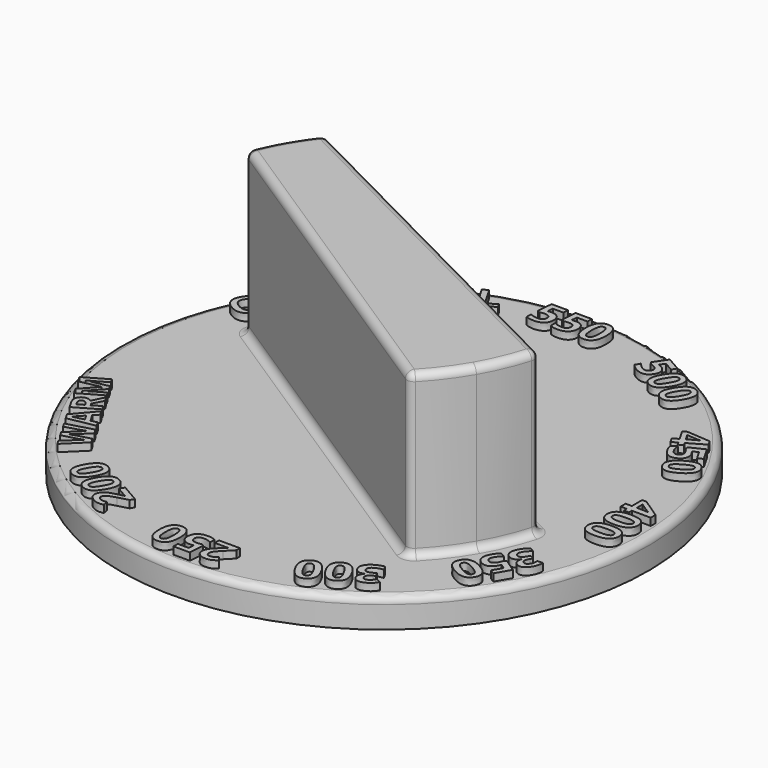
from build123d import *
from build123d import SkipClean  # not in build123d's __all__

# Parameters (mm, degrees)
F0_R          = 36
F0_R_2        = 5
F1_DEPTH      = 4
F2_DEPTH      = 26
F3_R          = 1
F4_DEPTH      = 25
F5_R          = 1
F6_DEPTH      = 4
F8_ANGLE      = -90
F9_TEXT_SIZE  = 5.2390307793
F10_DEPTH     = 1
F11_ANGLE     = 90
F12_TEXT_SIZE = 5.7419702135
F13_DEPTH     = 1
F14_ANGLE     = 30
F15_TEXT_SIZE = 5.7419702135
F16_DEPTH     = 1
F17_ANGLE     = 30
F18_TEXT_SIZE = 5.7419702135
F19_DEPTH     = 1
F20_ANGLE     = 30
F21_TEXT_SIZE = 5.7419702135
F22_DEPTH     = 1
F23_ANGLE     = 30
F24_TEXT_SIZE = 5.7419702135
F25_DEPTH     = 1
F26_ANGLE     = 30
F27_TEXT_SIZE = 5.7419702135
F28_DEPTH     = 1
F29_ANGLE     = 30
F30_TEXT_SIZE = 5.7419702135
F31_DEPTH     = 1
F32_ANGLE     = 60
F33_TEXT_SIZE = 5.2378516624
F34_DEPTH     = 1
F35_ANGLE     = 90
F36_TEXT_SIZE = 4.9233294015
F37_DEPTH     = 1
F38_ANGLE     = -120
F39_TEXT_SIZE = 5.7419702135
F40_DEPTH     = 1


# Not quite as in the source:
# - Text() gives the source's letters only with a copy of the font that has no kerning and outlines rounded to 1/6400 em; it was checked with that copy


with BuildPart() as f1:
    # F0 (on Top) → F1 (new body)
    with BuildSketch(Plane.XY):
        Circle(F0_R)
        with BuildLine():
            ThreePointArc((-26.2288567733, 6.6408985875), (-25.8537103282, 7.20647008), (-25.2038950976, 7.4022917703))
            Line((-25.2038950976, 7.4022917703), (27.7893484801, 4.5633680072))
            ThreePointArc((27.7893484801, 4.5633680072), (28.4145237228, 4.2992432559), (28.7270995296, 3.6968294999))
            ThreePointArc((28.7270995296, 3.6968294999), (28.9108711387, 1.8524734404), (28.9722179472, 0))
            ThreePointArc((28.9722179472, 0), (28.9108711387, -1.8524734404), (28.7270995296, -3.6968294999))
            ThreePointArc((28.7270995296, -3.6968294999), (28.4145237228, -4.2992432559), (27.7893484801, -4.5633680072))
            Line((27.7893484801, -4.5633680072), (-25.2038950976, -7.4022917703))
            ThreePointArc((-25.2038950976, -7.4022917703), (-25.8537103282, -7.20647008), (-26.2288567733, -6.6408985875))
            ThreePointArc((-26.2288567733, -6.6408985875), (-26.8273332377, -3.3443914115), (-27.0277820528, 0))
            ThreePointArc((-27.0277820528, 0), (-26.8273332377, 3.3443914115), (-26.2288567733, 6.6408985875))
        make_face(mode=Mode.SUBTRACT)
        with BuildLine():
            Line((27.7893484801, 4.5633680072), (-25.2038950976, 7.4022917703))
            ThreePointArc((-25.2038950976, 7.4022917703), (-25.8537103282, 7.20647008), (-26.2288567733, 6.6408985875))
            ThreePointArc((-26.2288567733, 6.6408985875), (-26.8273332377, 3.3443914115), (-27.0277820528, 0))
            ThreePointArc((-27.0277820528, 0), (-26.8273332377, -3.3443914115), (-26.2288567733, -6.6408985875))
            ThreePointArc((-26.2288567733, -6.6408985875), (-25.8537103282, -7.20647008), (-25.2038950976, -7.4022917703))
            Line((-25.2038950976, -7.4022917703), (27.7893484801, -4.5633680072))
            ThreePointArc((27.7893484801, -4.5633680072), (28.4145237228, -4.2992432559), (28.7270995296, -3.6968294999))
            ThreePointArc((28.7270995296, -3.6968294999), (28.9108711387, -1.8524734404), (28.9722179472, 0))
            ThreePointArc((28.9722179472, 0), (28.9108711387, 1.8524734404), (28.7270995296, 3.6968294999))
            ThreePointArc((28.7270995296, 3.6968294999), (28.4145237228, 4.2992432559), (27.7893484801, 4.5633680072))
        make_face()
        Circle(F0_R_2, mode=Mode.SUBTRACT)
        Circle(F0_R_2)
        with BuildLine():
            ThreePointArc((2.2360679775, 2), (0, -3), (-2.2360679775, 2))
            Line((-2.2360679775, 2), (2.2360679775, 2))
        make_face(mode=Mode.SUBTRACT)
        with BuildLine():
            Line((2.2360679775, 2), (-2.2360679775, 2))
            ThreePointArc((-2.2360679775, 2), (0, -3), (2.2360679775, 2))
        make_face()
    extrude(amount=F1_DEPTH)

    # F0 (on Top) → F2 (join)
    with BuildSketch(Plane.XY):
        with BuildLine():
            Line((27.7893484801, 4.5633680072), (-25.2038950976, 7.4022917703))
            ThreePointArc((-25.2038950976, 7.4022917703), (-25.8537103282, 7.20647008), (-26.2288567733, 6.6408985875))
            ThreePointArc((-26.2288567733, 6.6408985875), (-26.8273332377, 3.3443914115), (-27.0277820528, 0))
            ThreePointArc((-27.0277820528, 0), (-26.8273332377, -3.3443914115), (-26.2288567733, -6.6408985875))
            ThreePointArc((-26.2288567733, -6.6408985875), (-25.8537103282, -7.20647008), (-25.2038950976, -7.4022917703))
            Line((-25.2038950976, -7.4022917703), (27.7893484801, -4.5633680072))
            ThreePointArc((27.7893484801, -4.5633680072), (28.4145237228, -4.2992432559), (28.7270995296, -3.6968294999))
            ThreePointArc((28.7270995296, -3.6968294999), (28.9108711387, -1.8524734404), (28.9722179472, 0))
            ThreePointArc((28.9722179472, 0), (28.9108711387, 1.8524734404), (28.7270995296, 3.6968294999))
            ThreePointArc((28.7270995296, 3.6968294999), (28.4145237228, 4.2992432559), (27.7893484801, 4.5633680072))
        make_face()
        Circle(F0_R_2, mode=Mode.SUBTRACT)
        Circle(F0_R_2)
        with BuildLine():
            ThreePointArc((2.2360679775, 2), (0, -3), (-2.2360679775, 2))
            Line((-2.2360679775, 2), (2.2360679775, 2))
        make_face(mode=Mode.SUBTRACT)
        with BuildLine():
            Line((2.2360679775, 2), (-2.2360679775, 2))
            ThreePointArc((-2.2360679775, 2), (0, -3), (2.2360679775, 2))
        make_face()
    extrude(amount=F2_DEPTH)

    # F3
    f3_edges = [f1.edges().sort_by_distance(p)[0] for p in [
        (1.292727, 5.98283, 26),
        (28.414524, 4.299243, 26),
        (1.292727, -5.98283, 26),
        (-25.85371, 7.20647, 26),
        (-27.027782, 0, 26),
        (-25.85371, -7.20647, 26),
        (28.414524, -4.299243, 26),
        (28.972218, 0, 26),
    ]]
    fillet(f3_edges, radius=F3_R)

    # F0 (on Top) → F4 (cut)
    with BuildSketch(Plane.XY):
        with BuildLine():
            Line((2.2360679775, 2), (-2.2360679775, 2))
            ThreePointArc((-2.2360679775, 2), (0, -3), (2.2360679775, 2))
        make_face()
    extrude(amount=F4_DEPTH, mode=Mode.SUBTRACT)

    # F5
    f5_edges = [f1.edges().sort_by_distance(p)[0] for p in [
        (-36, 0, 4),
        (-25.85371, 7.20647, 4),
        (-27.027782, 0, 4),
        (-25.85371, -7.20647, 4),
        (1.292727, -5.98283, 4),
        (28.414524, -4.299243, 4),
        (28.972218, 0, 4),
        (28.414524, 4.299243, 4),
        (1.292727, 5.98283, 4),
    ]]
    fillet(f5_edges, radius=F5_R)

    # F0 (on Top) → F6 (join)
    with BuildSketch(Plane.XY):
        Circle(F0_R_2)
        with BuildLine():
            ThreePointArc((2.2360679775, 2), (0, -3), (-2.2360679775, 2))
            Line((-2.2360679775, 2), (2.2360679775, 2))
        make_face(mode=Mode.SUBTRACT)
    with SkipClean():  # cleaning this boolean's faces spoils the solid; the shape is the same uncleaned
        extrude(amount=-F6_DEPTH)


with BuildPart() as f1_1:
    # F8: moved
    add(f1.part.rotate(Axis((0, 0, 37.6716628671), (0, 0, -1)), F8_ANGLE), clean=False)

    # F9 (on face) → F10 (join)
    with BuildSketch(Plane.XY.offset(4)):
        with Locations((-4.9426552728, 30.7683626071)):
            Text('OFF', F9_TEXT_SIZE, font='Open Sans', font_style=FontStyle.BOLD, text_align=(TextAlign.LEFT, TextAlign.BOTTOM))
    extrude(amount=F10_DEPTH)


with BuildPart() as f1_2:
    # F11: moved
    add(f1_1.part.rotate(Axis((0, 0, 37.6716628671), (0, 0, -1)), F11_ANGLE), clean=False)

    # F12 (on face) → F13 (join)
    with BuildSketch(Plane.XY.offset(4)):
        with Locations((-5, 30.3274479291)):
            Text('200', F12_TEXT_SIZE, font='Open Sans', font_style=FontStyle.BOLD, text_align=(TextAlign.LEFT, TextAlign.BOTTOM))
    extrude(amount=F13_DEPTH)


with BuildPart() as f1_3:
    # F14: moved
    add(f1_2.part.rotate(Axis((0, 0, 37.6716628671), (0, 0, -1)), F14_ANGLE), clean=False)

    # F15 (on face) → F16 (join)
    with BuildSketch(Plane.XY.offset(4)):
        with Locations((-5, 30.5067975976)):
            Text('250', F15_TEXT_SIZE, font='Open Sans', font_style=FontStyle.BOLD, text_align=(TextAlign.LEFT, TextAlign.BOTTOM))
    extrude(amount=F16_DEPTH)


with BuildPart() as f1_4:
    # F17: moved
    add(f1_3.part.rotate(Axis((0, 0, 37.6716628671), (0, 0, -1)), F17_ANGLE), clean=False)

    # F18 (on face) → F19 (join)
    with BuildSketch(Plane.XY.offset(4)):
        with Locations((-5, 30.5067975976)):
            Text('300', F18_TEXT_SIZE, font='Open Sans', font_style=FontStyle.BOLD, text_align=(TextAlign.LEFT, TextAlign.BOTTOM))
    extrude(amount=F19_DEPTH)


with BuildPart() as f1_5:
    # F20: moved
    add(f1_4.part.rotate(Axis((0, 0, 37.6716628671), (0, 0, -1)), F20_ANGLE), clean=False)

    # F21 (on face) → F22 (join)
    with BuildSketch(Plane.XY.offset(4)):
        with Locations((-5, 30.5067975976)):
            Text('350', F21_TEXT_SIZE, font='Open Sans', font_style=FontStyle.BOLD, text_align=(TextAlign.LEFT, TextAlign.BOTTOM))
    extrude(amount=F22_DEPTH)


with BuildPart() as f1_6:
    # F23: moved
    add(f1_5.part.rotate(Axis((0, 0, 37.6716628671), (0, 0, -1)), F23_ANGLE), clean=False)

    # F24 (on face) → F25 (join)
    with BuildSketch(Plane.XY.offset(4)):
        with Locations((-5, 30.4273520987)):
            Text('400', F24_TEXT_SIZE, font='Open Sans', font_style=FontStyle.BOLD, text_align=(TextAlign.LEFT, TextAlign.BOTTOM))
    extrude(amount=F25_DEPTH)


with BuildPart() as f1_7:
    # F26: moved
    add(f1_6.part.rotate(Axis((0, 0, 37.6716628671), (0, 0, -1)), F26_ANGLE), clean=False)

    # F27 (on face) → F28 (join)
    with BuildSketch(Plane.XY.offset(4)):
        with Locations((-5, 30.5067975976)):
            Text('450', F27_TEXT_SIZE, font='Open Sans', font_style=FontStyle.BOLD, text_align=(TextAlign.LEFT, TextAlign.BOTTOM))
    extrude(amount=F28_DEPTH)


with BuildPart() as f1_8:
    # F29: moved
    add(f1_7.part.rotate(Axis((0, 0, 37.6716628671), (0, 0, -1)), F29_ANGLE), clean=False)

    # F30 (on face) → F31 (join)
    with BuildSketch(Plane.XY.offset(4)):
        with Locations((-5, 30.3368268976)):
            Text('500', F30_TEXT_SIZE, font='Open Sans', font_style=FontStyle.BOLD, text_align=(TextAlign.LEFT, TextAlign.BOTTOM))
    extrude(amount=F31_DEPTH)


with BuildPart() as f1_9:
    # F32: moved
    add(f1_8.part.rotate(Axis((0, 0, 37.6716628671), (0, 0, -1)), F32_ANGLE), clean=False)

    # F33 (on face) → F34 (join)
    with BuildSketch(Plane.XY.offset(4)):
        with Locations((-8, 30.3021968779)):
            Text('BROIL', F33_TEXT_SIZE, font='Open Sans', font_style=FontStyle.BOLD, text_align=(TextAlign.LEFT, TextAlign.BOTTOM))
    extrude(amount=F34_DEPTH)


with BuildPart() as f1_10:
    # F35: moved
    add(f1_9.part.rotate(Axis((0, 0, 37.6716628671), (0, 0, -1)), F35_ANGLE), clean=False)

    # F36 (on face) → F37 (join)
    with BuildSketch(Plane.XY.offset(4)):
        with Locations((-7.9631006718, 30.4550943151)):
            Text('WARM', F36_TEXT_SIZE, font='Open Sans', font_style=FontStyle.BOLD, text_align=(TextAlign.LEFT, TextAlign.BOTTOM))
    extrude(amount=F37_DEPTH)


with BuildPart() as f1_11:
    # F38: moved
    add(f1_10.part.rotate(Axis((0, 0, 37.6716628671), (0, 0, -1)), F38_ANGLE), clean=False)

    # F39 (on face) → F40 (join)
    with BuildSketch(Plane.XY.offset(4)):
        with Locations((-5, 30.0628316097)):
            Text('550', F39_TEXT_SIZE, font='Open Sans', font_style=FontStyle.BOLD, text_align=(TextAlign.LEFT, TextAlign.BOTTOM))
    extrude(amount=F40_DEPTH)


solid = f1_11.part
